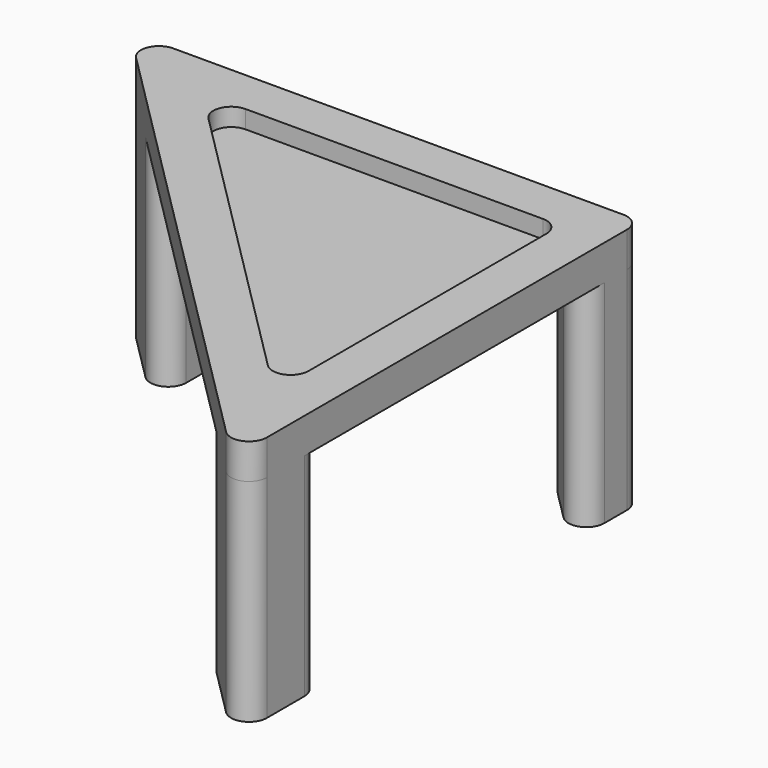
from build123d import *

# Parameters (mm, degrees)
F1_DEPTH = 10
F2_R     = 5.08
F4_DEPTH = 60
F5_R     = 5.08
F7_DEPTH = 5.08
F8_R     = 5.08


# Not quite as in the source:
# - a feature names something its author has since deleted; it is built from what else it names


with BuildPart() as f1:
    # F0 (on Top) → F1 (new body)
    with BuildSketch(Plane.XY):
        Polygon((63.5, 38.1), (63.5, 63.5), (38.1, 63.5), (50.8, 50.8), align=None)
        Polygon((50.8, 50.8), (38.1, 63.5), (-50.8, 63.5), (-50.8, 32.8394877579), (32.8394877579, -50.8), (63.5, -50.8), (63.5, 38.1), align=None)
        Polygon((-50.8, 32.8394877579), (-50.8, 63.5), (-81.4605122421, 63.5), align=None)
        Polygon((63.5, -81.4605122421), (63.5, -50.8), (32.8394877579, -50.8), align=None)
    extrude(amount=F1_DEPTH)

    # F2
    f2_edges = [f1.edges().sort_by_distance(p)[0] for p in [
        (63.5, -81.460512, 5),
        (-81.460512, 63.5, 5),
        (63.5, 63.5, 5),
    ]]
    fillet(f2_edges, radius=F2_R)

    # F0 (on Top) + F3 (on face) → F4 (join)
    with BuildSketch(Plane.XY):
        Polygon((63.5, -81.4605122421), (63.5, -50.8), (32.8394877579, -50.8), align=None)
        Polygon((63.5, 38.1), (63.5, 63.5), (38.1, 63.5), (50.8, 50.8), align=None)
    with BuildSketch(Plane.XY):
        Polygon((-50.8, 63.5), (-81.4605122421, 63.5), (-50.8, 32.8394877579), align=None)
    extrude(amount=-F4_DEPTH)

    # F5
    f5_edges = [f1.edges().sort_by_distance(p)[0] for p in [
        (-81.460512, 63.5, -30),
        (63.5, -81.460512, -30),
        (63.5, 63.5, -30),
        (32.839488, -50.8, -30),
        (-50.8, 32.839488, -30),
        (-50.8, 63.5, -30),
        (38.1, 63.5, -30),
        (63.5, 38.1, -30),
        (63.5, -50.8, -30),
    ]]
    fillet(f5_edges, radius=F5_R)

    # F6 (on face) → F7 (cut)
    with BuildSketch(Plane.XY.offset(10)):
        Polygon((50.8, 50.8), (-50.8, 50.8), (50.8, -50.8), align=None)
    extrude(amount=-F7_DEPTH, mode=Mode.SUBTRACT)

    # F8
    f8_edges = [f1.edges().sort_by_distance(p)[0] for p in [
        (50.8, 50.8, 7.46),
        (-50.8, 50.8, 7.46),
        (50.8, -50.8, 7.46),
    ]]
    fillet(f8_edges, radius=F8_R)


solid = f1.part
